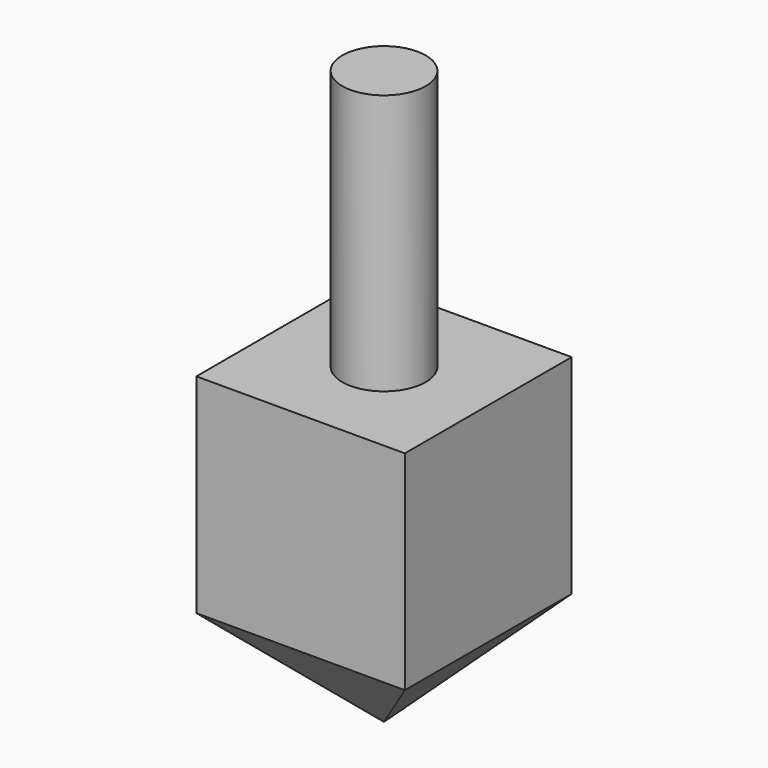
from build123d import *

# Parameters (mm, degrees)
F0_W     = 20
F0_H     = 20
F1_DEPTH = 30
F2_R     = 4
F3_DEPTH = 25
F4_SIZE  = 9.99999


# Not quite as in the source:
# - a fillet or chamfer is up to 0.001 mm smaller than in the source, because OpenCascade refuses the exact size


with BuildPart() as f1:
    # F0 (on Top) → F1 (new body)
    with BuildSketch(Plane.XY):
        Rectangle(F0_W, F0_H)
    extrude(amount=F1_DEPTH)

    # F2 (on face) → F3 (join)
    with BuildSketch(Plane.XY.offset(30)):
        Circle(F2_R)
    extrude(amount=F3_DEPTH)

    # F4 (size 10 in the source; OpenCascade refuses exactly that, so slightly less here)
    f4_edges = [f1.edges().sort_by_distance(p)[0] for p in [
        (10, 0, 0),
        (0, 10, 0),
        (-10, 0, 0),
        (0, -10, 0),
    ]]
    chamfer(f4_edges, length=F4_SIZE)


solid = f1.part
